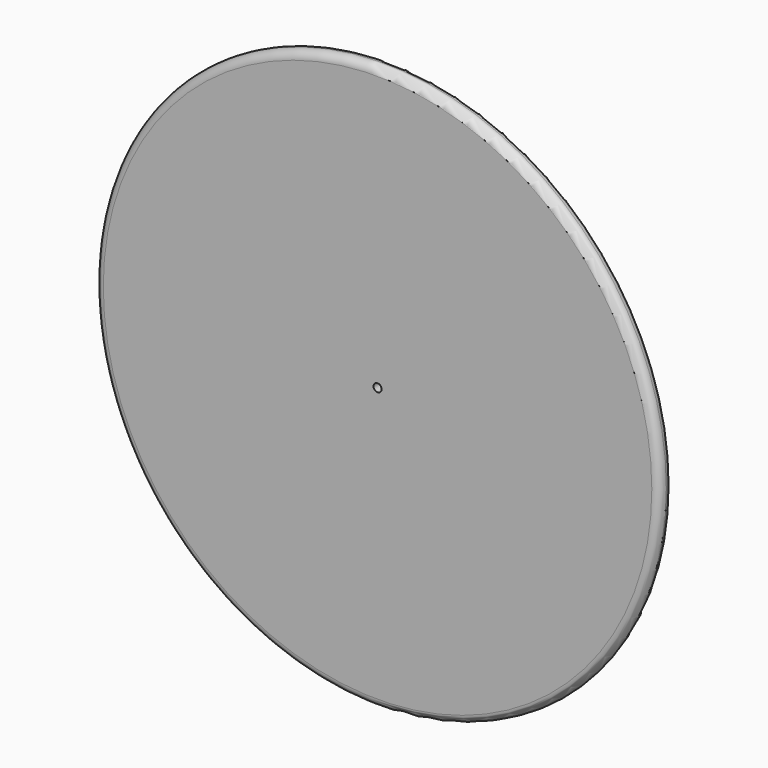
from build123d import *

# Parameters (mm, degrees)
F0_R     = 88.9
F0_R_2   = 1.27
F1_DEPTH = 5.08
F2_R     = 2.53999


# Not quite as in the source:
# - a fillet or chamfer is up to 0.001 mm smaller than in the source, because OpenCascade refuses the exact size


with BuildPart() as f1:
    # F0 (on Front) → F1 (new body)
    with BuildSketch(Plane.XZ):
        Circle(F0_R)
        Circle(F0_R_2, mode=Mode.SUBTRACT)
    extrude(amount=F1_DEPTH)

    # F2 (radius 2.54 in the source; OpenCascade refuses exactly that, so slightly less here)
    f2_edges = [f1.edges().sort_by_distance(p)[0] for p in [
        (-88.9, -5.08, 0),
        (-88.9, 0, 0),
    ]]
    fillet(f2_edges, radius=F2_R)


solid = f1.part
